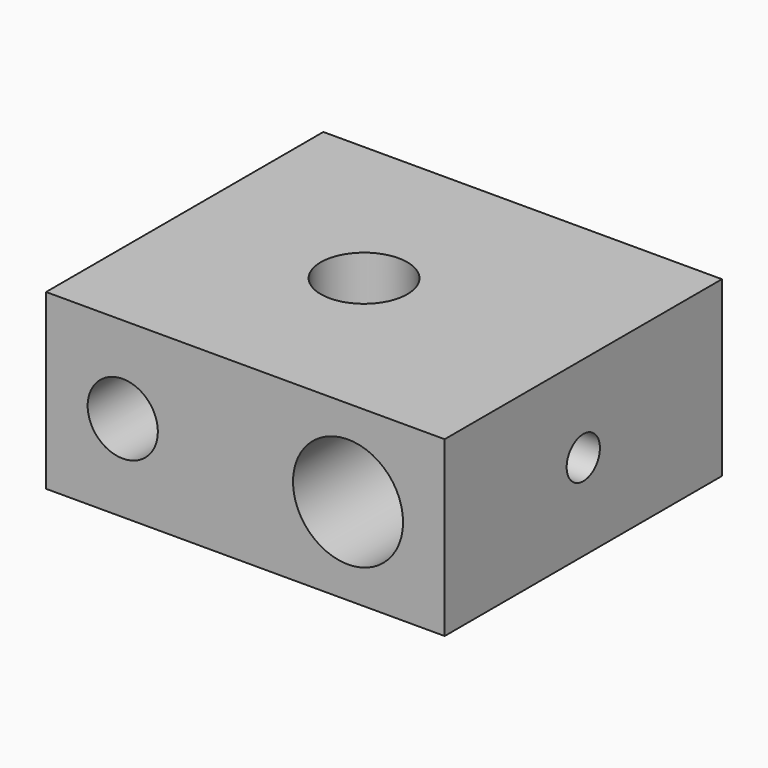
from build123d import *

# Parameters (mm, degrees)
F0_W     = 23
F0_H     = 20
F1_DEPTH = 5
F2_R     = 2.025
F2_R_2   = 3.175
F3_DEPTH = 25
F5_D     = 5
F7_D     = 2.4
F7_DEPTH = 5
F7_TIP   = 0.7210327428
F9_D     = 2.4
F9_DEPTH = 5
F9_TIP   = 0.7210327428


with BuildPart() as f1:
    # F0 (on Top) → F1 (new body, symmetric)
    with BuildSketch(Plane.XY):
        Rectangle(F0_W, F0_H)
    extrude(amount=F1_DEPTH, both=True)

    # F2 (on face) → F3 (cut)
    with BuildSketch(Plane.XZ.offset(10)):
        with Locations((-7.075, 0)):
            Circle(F2_R)
        with Locations((5.925, 0)):
            Circle(F2_R_2)
    extrude(amount=-F3_DEPTH, mode=Mode.SUBTRACT)

    # F5 (through all)
    with Locations(Plane.XY.offset(5)):
        with Locations((-1.15, 0)):
            Hole(F5_D / 2)

    # F7
    with Locations(Plane(origin=(-11.5, 0, 0), x_dir=(0, -1, 0), z_dir=(-1, 0, 0))):
        with Locations((0, 0)):
            Hole(F7_D / 2, depth=F7_DEPTH)
            with Locations((0, 0, -(F7_DEPTH + F7_TIP / 2))):  # 118° drill point
                Cone(0, F7_D / 2, F7_TIP, mode=Mode.SUBTRACT)

    # F9
    with Locations(Plane.YZ.offset(11.5)):
        with Locations((0, 0)):
            Hole(F9_D / 2, depth=F9_DEPTH)
            with Locations((0, 0, -(F9_DEPTH + F9_TIP / 2))):  # 118° drill point
                Cone(0, F9_D / 2, F9_TIP, mode=Mode.SUBTRACT)


solid = f1.part
